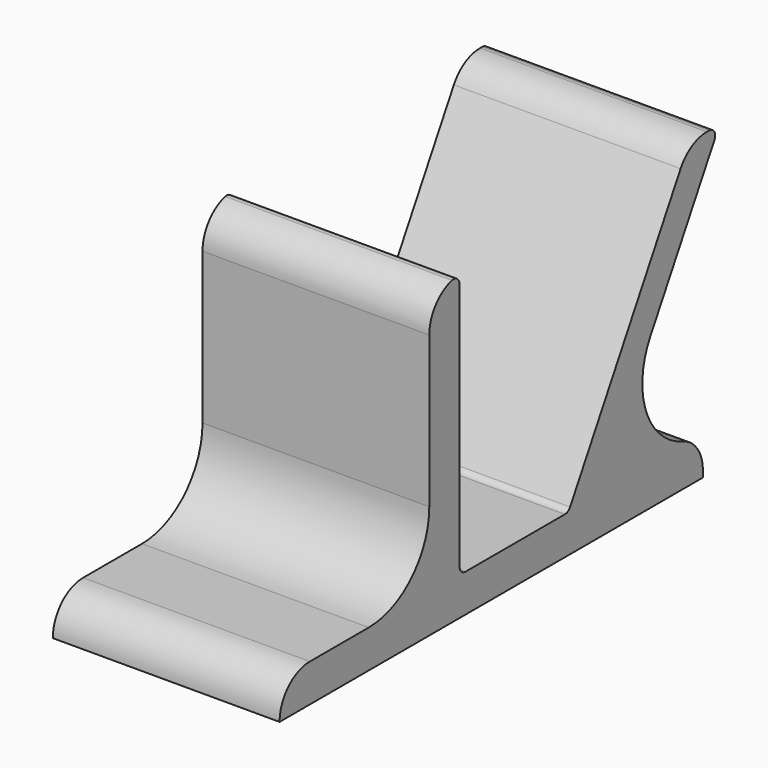
from build123d import *

# Parameters (mm, degrees)
F1_DEPTH    = 30
F2_R        = 10
F3_T1_DEPTH = 56.2345635929
F3_T3_DEPTH = 50.7373541457
F3_T5_DEPTH = 44.5080633868
F3_T7_DEPTH = 55
F4_R        = 1


# Not quite as in the source:
# - a fillet or chamfer that OpenCascade refuses, or shapes differently, is made with other operations: its cross-section is extruded or revolved along the edge and cut away or added


with BuildPart() as f1:
    # F0 (on Right) → F1 (new body)
    with BuildSketch(Plane.YZ):
        Polygon((-27.3037352718, 5), (-27.0568225533, 0), (42.9431774467, 0), (42.9431774467, 5), (25.6962647282, 5), (45.6962647282, 40), (40.6962647282, 40), (20.6962647282, 5), (8.8888889937, 5), (2.6962647282, 5), (2.6962647282, 40), (-2.3037352718, 40), (-2.3037352718, 5), align=None)
    extrude(amount=F1_DEPTH)

    # F2
    f2_edges = [f1.edges().sort_by_distance(p)[0] for p in [
        (15, 25.696265, 5),
        (15, -2.303735, 5),
    ]]
    fillet(f2_edges, radius=F2_R)

    # F3: fillet of radius 5 on 4 edges, made by hand

    # F3_s2 → F3_t1 (cut)
    with BuildSketch(Plane.YZ.offset(-13.1172817964)):
        with BuildLine():
            ThreePointArc((-22.0568225533, 5), (-25.5923564592, 3.5355339059), (-27.0568225533, 0))
            Line((-27.0568225533, 0), (-27.3037352718, 5))
            Line((-27.3037352718, 5), (-22.0568225533, 5))
        make_face()
    extrude(amount=F3_T1_DEPTH, mode=Mode.SUBTRACT)

    # F3_s4 → F3_t3 (cut)
    with BuildSketch(Plane.YZ.offset(-10.3686770729)):
        with BuildLine():
            ThreePointArc((42.9431774467, 0.8525291709), (42.0241172961, 3.7414614903), (39.6048054683, 5.5683527806))
            Line((39.6048054683, 5.5683527806), (39.7709682705, 6.0399351415))
            ThreePointArc((39.7709682705, 6.0399351415), (42.9280615114, 5.5), (42.9431774467, 5.5))
            Line((42.9431774467, 5.5), (43.4431774467, 5))
            Line((43.4431774467, 5), (43.4431774467, 0.8525291709))
            Line((43.4431774467, 0.8525291709), (42.9431774467, 0.8525291709))
        make_face()
    extrude(amount=F3_T3_DEPTH, mode=Mode.SUBTRACT)

    # F3_s6 → F3_t5 (cut)
    with BuildSketch(Plane.YZ.offset(-7.2540316934)):
        with BuildLine():
            ThreePointArc((39.2566616949, 37.4806946918), (41.0882433145, 39.3245504656), (43.5978774055, 40))
            Line((43.5978774055, 40), (40.6962647282, 40))
            Line((40.6962647282, 40), (39.2566616949, 37.4806946918))
        make_face()
    extrude(amount=F3_T5_DEPTH, mode=Mode.SUBTRACT)

    # F3_s8 → F3_t7 (cut)
    with BuildSketch(Plane.YZ.offset(-12.5)):
        with BuildLine():
            ThreePointArc((-2.3037352718, 35), (-0.8392691778, 38.5355339059), (2.6962647282, 40))
            Line((2.6962647282, 40), (-2.3037352718, 40))
            Line((-2.3037352718, 40), (-2.3037352718, 35))
        make_face()
    extrude(amount=F3_T7_DEPTH, mode=Mode.SUBTRACT)

    # F4
    f4_edges = [f1.edges().sort_by_distance(p)[0] for p in [
        (15, 2.696265, 5),
        (15, 20.696265, 5),
        (15, 2.696265, 40),
        (15, 45.696265, 40),
    ]]
    fillet(f4_edges, radius=F4_R)


solid = f1.part
